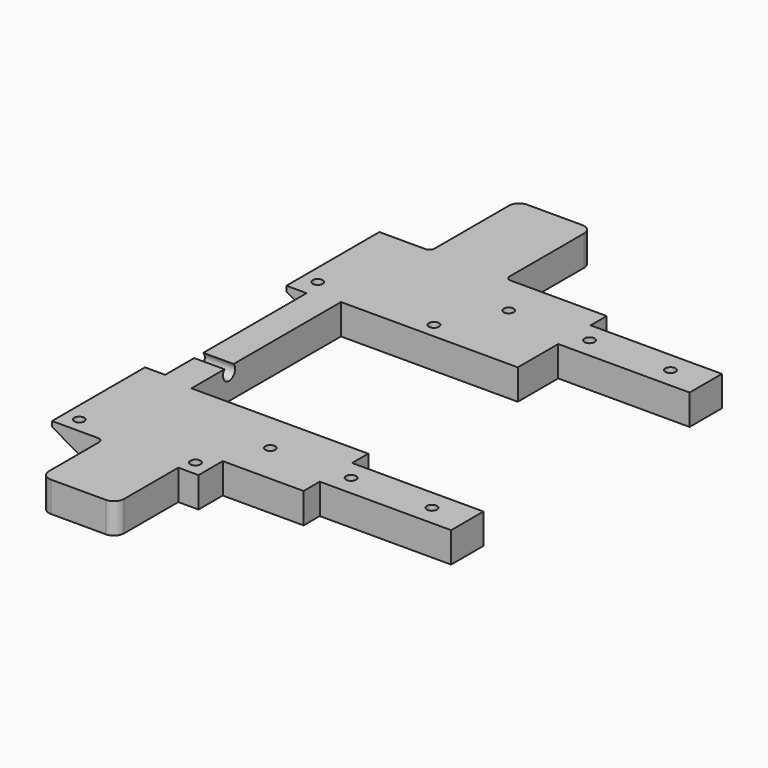
from build123d import *

# Parameters (mm, degrees)
F0_R     = 3.175
F1_DEPTH = 19.05
F2_R     = 4.7879
F3_DEPTH = 50.8
F5_DEPTH = 279.4


# Not quite as in the source:
# - a feature names something its author has since deleted; it is built from what else it names


with BuildPart() as f1:
    # F0 (on Top) → F1 (new body)
    with BuildSketch(Plane.XY):
        with BuildLine():
            Line((-118.9269337424, 53.8231658584), (-147.8829337424, 53.8231658584))
            Line((-147.8829337424, 53.8231658584), (-147.8829337424, -16.0268341416))
            Line((-147.8829337424, -16.0268341416), (-147.8829337424, -19.2018341416))
            Line((-147.8829337424, -19.2018341416), (-135.1829337424, -19.2018341416))
            Line((-135.1829337424, -19.2018341416), (-135.1829337424, -130.3268341416))
            Line((-135.1829337424, -130.3268341416), (-147.8829337424, -130.3268341416))
            Line((-147.8829337424, -130.3268341416), (-147.8829337424, -136.6768341416))
            Line((-147.8829337424, -136.6768341416), (-147.8829337424, -171.6018341416))
            Line((-147.8829337424, -171.6018341416), (-147.8829337424, -203.3518341416))
            Line((-147.8829337424, -203.3518341416), (-118.9269337424, -203.3518341416))
            ThreePointArc((-118.9269337424, -203.3518341416), (-116.6818697121, -204.2817701113), (-115.7519337424, -206.5268341416))
            Line((-115.7519337424, -206.5268341416), (-115.7519337424, -245.9476341416))
            ThreePointArc((-115.7519337424, -245.9476341416), (-113.8920618029, -250.4377622021), (-109.4019337424, -252.2976341416))
            Line((-109.4019337424, -252.2976341416), (-74.8579337424, -252.2976341416))
            ThreePointArc((-74.8579337424, -252.2976341416), (-70.3678056819, -250.4377622021), (-68.5079337424, -245.9476341416))
            Line((-68.5079337424, -245.9476341416), (-68.5079337424, -203.3518341416))
            Line((-68.5079337424, -203.3518341416), (-55.8079337424, -203.3518341416))
            Line((-55.8079337424, -203.3518341416), (-55.8079337424, -184.3018341416))
            Line((-55.8079337424, -184.3018341416), (-5.0079337424, -184.3018341416))
            Line((-5.0079337424, -184.3018341416), (-5.0079337424, -171.6018341416))
            Line((-5.0079337424, -171.6018341416), (77.5420662576, -171.6018341416))
            Line((77.5420662576, -171.6018341416), (77.5420662576, -146.2018341416))
            Line((77.5420662576, -146.2018341416), (-5.0079337424, -146.2018341416))
            Line((-5.0079337424, -146.2018341416), (-5.0079337424, -133.5018341416))
            Line((-5.0079337424, -133.5018341416), (-27.2329337424, -133.5018341416))
            Line((-27.2329337424, -133.5018341416), (-116.1329337424, -133.5018341416))
            Line((-116.1329337424, -133.5018341416), (-116.1329337424, -16.0268341416))
            Line((-116.1329337424, -16.0268341416), (-22.9684459845, -16.0268341416))
            Line((-22.9684459845, -16.0268341416), (-5.0079337424, -16.0268341416))
            Line((-5.0079337424, -16.0268341416), (-5.0079337424, -7.9982466186))
            Line((-5.0079337424, -7.9982466186), (-5.0079337424, 15.7231658584))
            Line((-5.0079337424, 15.7231658584), (77.5420662576, 15.7231658584))
            Line((77.5420662576, 15.7231658584), (77.5420662576, 41.1231658584))
            Line((77.5420662576, 41.1231658584), (-5.0079337424, 41.1231658584))
            Line((-5.0079337424, 41.1231658584), (-5.0079337424, 53.8231658584))
            Line((-5.0079337424, 53.8231658584), (-65.3329337424, 53.8231658584))
            ThreePointArc((-65.3329337424, 53.8231658584), (-67.5779977727, 54.7531018282), (-68.5079337424, 56.9981658584))
            Line((-68.5079337424, 56.9981658584), (-68.5079337424, 115.4689658584))
            ThreePointArc((-68.5079337424, 115.4689658584), (-70.3678056819, 119.959093919), (-74.8579337424, 121.8189658584))
            Line((-74.8579337424, 121.8189658584), (-109.4019337424, 121.8189658584))
            ThreePointArc((-109.4019337424, 121.8189658584), (-113.8920618029, 119.959093919), (-115.7519337424, 115.4689658584))
            Line((-115.7519337424, 115.4689658584), (-115.7519337424, 56.9981658584))
            ThreePointArc((-115.7519337424, 56.9981658584), (-116.6818697121, 54.7531018282), (-118.9269337424, 53.8231658584))
        make_face()
        with Locations((-138.3579337424, -193.8268341416)):
            Circle(F0_R, mode=Mode.SUBTRACT)
        with Locations((-65.3329337424, -193.8268341416)):
            Circle(F0_R, mode=Mode.SUBTRACT)
        with Locations((-46.2829337424, -158.9018341416)):
            Circle(F0_R, mode=Mode.SUBTRACT)
        with Locations((4.5170662576, -158.9018341416)):
            Circle(F0_R, mode=Mode.SUBTRACT)
        with Locations((55.3170662576, -158.9018341416)):
            Circle(F0_R, mode=Mode.SUBTRACT)
        with Locations((-138.3579337424, -6.5018341416)):
            Circle(F0_R, mode=Mode.SUBTRACT)
        with Locations((-65.3329337424, -6.5018341416)):
            Circle(F0_R, mode=Mode.SUBTRACT)
        with Locations((-46.2829337424, 28.4231658584)):
            Circle(F0_R, mode=Mode.SUBTRACT)
        with Locations((4.5170662576, 28.4231658584)):
            Circle(F0_R, mode=Mode.SUBTRACT)
        with Locations((55.3170662576, 28.4231658584)):
            Circle(F0_R, mode=Mode.SUBTRACT)
    extrude(amount=F1_DEPTH)

    # F2 (on face) → F3 (cut)
    with BuildSketch(Plane(origin=(-147.8829337424, 0, 0), x_dir=(0, -1, 0), z_dir=(-1, 0, 0))):
        with Locations((103.9362341416, 15.875)):
            Circle(F2_R)
    extrude(amount=-F3_DEPTH, mode=Mode.SUBTRACT)

    # F4 (on face) → F5 (cut)
    with BuildSketch(Plane.XZ.offset(203.3518341416)):
        Polygon((-120.3866271722, 0), (-147.8829337424, 15.875), (-147.8829337424, 0), align=None)
    extrude(amount=-F5_DEPTH, mode=Mode.SUBTRACT)


solid = f1.part
